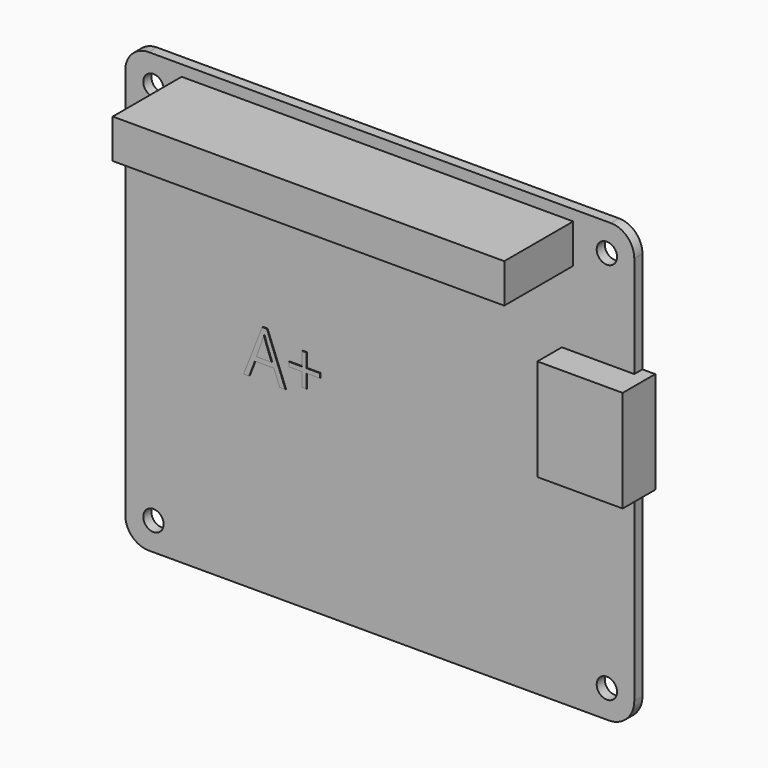
from build123d import *

# Parameters (mm, degrees)
F0_R         = 1.3
F0_W         = 50
F0_H         = 5
F1_DEPTH     = 1.3
F2_DEPTH     = 12.3
F0_W_2       = 9.25
F0_H_2       = 13
F0_W_3       = 1.64
F3_DEPTH     = 5.2
F0_TEXT_SIZE = 8.4436246349
F4_DEPTH     = 1.4
F5_DEPTH     = 1.5


# Not quite as in the source:
# - ends of sketch curves that miss each other by under 0.0002 mm in the source are joined
# - Text() gives the source's letters only with a copy of the font that has no kerning and outlines rounded to 1/6400 em; it was checked with that copy


with BuildPart() as f1:
    # F0 (on Front) → F1 (new body)
    with BuildSketch(Plane.XZ):
        with BuildLine():
            Line((31.8453074208, 21.0069748506), (31.8453074208, 21.558403905))
            ThreePointArc((31.8453074208, 21.558403905), (30.9671330716, 23.679218821), (28.8467368156, 24.5584035645))
            Line((28.8467368156, 24.5584035645), (-30.1532529376, 24.5865149939))
            ThreePointArc((-30.1532529376, 24.5865149939), (-32.2754972484, 23.7083409852), (-33.1546823324, 21.5865153344))
            Line((-33.1546823324, 21.5865153344), (-33.154689282, -28.4430251494))
            ThreePointArc((-33.154689282, -28.4430251494), (-32.2760096255, -30.564345493), (-30.154689282, -31.4430251494))
            Line((-30.154689282, -31.4430251494), (28.595300474, -31.4430251494))
            ThreePointArc((28.595300474, -31.4430251494), (30.893402425, -30.4911201536), (31.8453074208, -28.1930182026))
            Line((31.8453074208, -28.1930182026), (31.8453074208, -4.4430251494))
            Line((31.8453074208, -4.4430251494), (22.5953074208, -4.4430251494))
            Line((22.5953074208, -4.4430251494), (22.5953074208, 8.5569748506))
            Line((22.5953074208, 8.5569748506), (31.8453074208, 8.5569748506))
            Line((31.8453074208, 8.5569748506), (31.8453074208, 21.0069748506))
        make_face()
        with Locations((-29.554689282, -27.8734850061)):
            Circle(F0_R, mode=Mode.SUBTRACT)
        Polygon((-12.6195598114, -7.5961076654), (-13.3451838034, -7.5961076654), (-14.0958748061, -5.6791410101), (-16.5115430415, -5.6791410101), (-17.2529988298, -7.5961076654), (-17.9627910256, -7.5961076654), (-15.580105699, -1.5430842553), (-14.9903712909, -1.5430842553), align=None, mode=Mode.SUBTRACT)
        Polygon((-9.9268351426, -2.5708316913), (-9.9268351426, -4.3347576502), (-8.2288750012, -4.3347576502), (-8.2288750012, -4.9033829967), (-9.9268351426, -4.9033829967), (-9.9268351426, -6.6607123739), (-10.5007377545, -6.6607123739), (-10.5007377545, -4.9033829967), (-12.1907819979, -4.9033829967), (-12.1907819979, -4.3347576502), (-10.5007377545, -4.3347576502), (-10.5007377545, -2.5708316913), align=None, mode=Mode.SUBTRACT)
        with Locations((28.3453074208, -27.8930251494)):
            Circle(F0_R, mode=Mode.SUBTRACT)
        with Locations((-29.554689282, 21.0265149939)):
            Circle(F0_R, mode=Mode.SUBTRACT)
        with Locations((-0.9546926388, 20.6826181536)):
            Rectangle(F0_W, F0_H, mode=Mode.SUBTRACT)
        with Locations((28.3453074208, 21.0069748506)):
            Circle(F0_R, mode=Mode.SUBTRACT)
    extrude(amount=F1_DEPTH)

    # F0 (on Front) → F2 (join)
    with BuildSketch(Plane.XZ):
        with Locations((-0.9546926388, 20.6826181536)):
            Rectangle(F0_W, F0_H)
    extrude(amount=F2_DEPTH)

    # F0 (on Front) → F3 (join)
    with BuildSketch(Plane.XZ):
        with Locations((27.2203074208, 2.0569748506)):
            Rectangle(F0_W_2, F0_H_2)
        with Locations((32.6653074208, 2.0569748506)):
            Rectangle(F0_W_3, F0_H_2)
    extrude(amount=F3_DEPTH)

    # F0 (on Front) → F4 (join)
    with BuildSketch(Plane.XZ):
        with BuildLine():
            Line((-16.2635115679, -5.0485077951), (-14.3135620037, -5.0485077951))
            Line((-14.3135620037, -5.0485077951), (-15.0154383015, -3.1803558447))
            add(Edge.make_bspline(
                [(-15.0154383015, -3.1803558447), (-15.1513278855, -2.8254597467), (-15.2951333675, -2.3109263705)],
                knots=[0, 0, 0, 1, 1, 1], degree=2))
            add(Edge.make_bspline(
                [(-15.2951333675, -2.3109263705), (-15.3861661956, -2.7067212753), (-15.5550386883, -3.1803558447)],
                knots=[0, 0, 0, 1, 1, 1], degree=2))
            Line((-15.5550386883, -3.1803558447), (-16.2635115679, -5.0485077951))
        make_face()
        with Locations((-17.9627910256, -7.5961076654)):
            Text('A+', F0_TEXT_SIZE, font='Open Sans', text_align=(TextAlign.LEFT, TextAlign.BOTTOM))
    extrude(amount=F4_DEPTH)

    # F0 (on Front) → F5 (join)
    with BuildSketch(Plane.XZ):
        with BuildLine():
            Line((-16.2635115679, -5.0485077951), (-14.3135620037, -5.0485077951))
            Line((-14.3135620037, -5.0485077951), (-15.0154383015, -3.1803558447))
            add(Edge.make_bspline(
                [(-15.0154383015, -3.1803558447), (-15.1513278855, -2.8254597467), (-15.2951333675, -2.3109263705)],
                knots=[0, 0, 0, 1, 1, 1], degree=2))
            add(Edge.make_bspline(
                [(-15.2951333675, -2.3109263705), (-15.3861661956, -2.7067212753), (-15.5550386883, -3.1803558447)],
                knots=[0, 0, 0, 1, 1, 1], degree=2))
            Line((-15.5550386883, -3.1803558447), (-16.2635115679, -5.0485077951))
        make_face()
    extrude(amount=F5_DEPTH)


solid = f1.part
